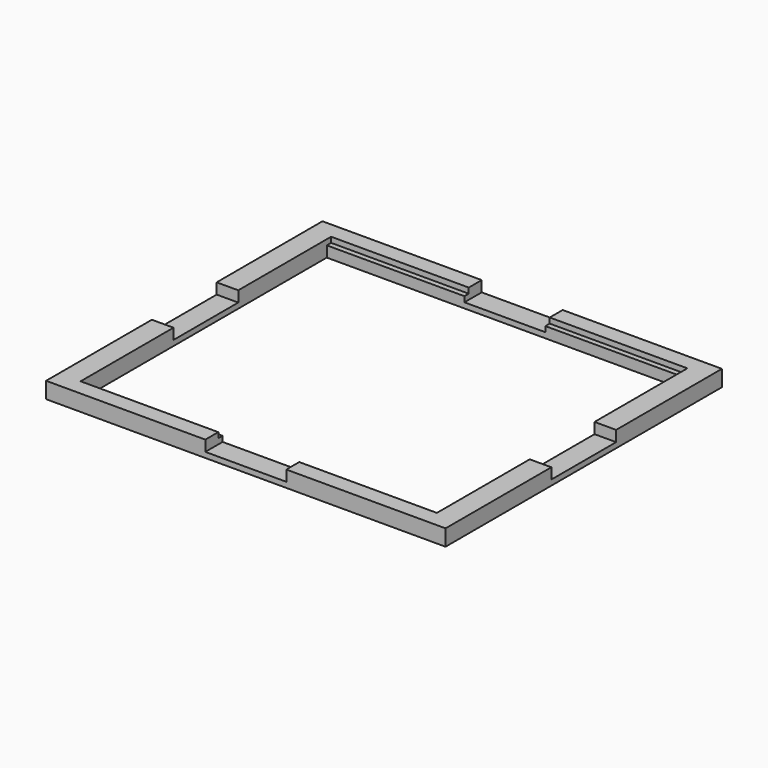
from build123d import *

# Parameters (mm, degrees)
F0_W     = 74
F0_H     = 64
F0_W_2   = 68
F0_H_2   = 58
F0_W_3   = 66
F0_H_3   = 56
F1_DEPTH = 2
F2_W     = 74
F2_H     = 64
F3_DEPTH = 1
F4_W     = 15
F4_H     = 6.5584733043
F4_H_2   = 3
F4_H_3   = 6.1532862581
F4_W_2   = 4
F4_H_4   = 15
F4_W_3   = 1.5584733043
F4_W_4   = 10.1532862581
F5_DEPTH = 2


with BuildPart() as f1:
    # F0 (on Top) → F1 (new body)
    with BuildSketch(Plane.XY):
        with Locations((-34, -29)):
            Rectangle(F0_W, F0_H)
        with Locations((-34, -29)):
            Rectangle(F0_W_2, F0_H_2, mode=Mode.SUBTRACT)
        with Locations((-34, -29)):
            Rectangle(F0_W_2, F0_H_2)
        with Locations((-34, -29)):
            Rectangle(F0_W_3, F0_H_3, mode=Mode.SUBTRACT)
    extrude(amount=F1_DEPTH)

    # F2 (on face) → F3 (join)
    with BuildSketch(Plane.XY.offset(2)):
        with Locations((-34, -29)):
            Rectangle(F2_W, F2_H)
        Polygon((-67, 0), (-1, 0), (-1, -1), (-1, -57), (-1, -58), (-67, -58), (-67, -57), (-67, -1), align=None, mode=Mode.SUBTRACT)
    extrude(amount=F3_DEPTH)

    # F4 (on face) → F5 (cut)
    with BuildSketch(Plane.XY.offset(3)):
        with Locations((-34, 6.2792366521)):
            Rectangle(F4_W, F4_H)
        with Locations((-34, 1.5)):
            Rectangle(F4_W, F4_H_2)
        with Locations((-34, -3.0766431291)):
            Rectangle(F4_W, F4_H_3)
        with Locations((1, -29)):
            Rectangle(F4_W_2, F4_H_4)
        with Locations((3.7792366521, -29)):
            Rectangle(F4_W_3, F4_H_4)
        with Locations((-6.0766431291, -29)):
            Rectangle(F4_W_4, F4_H_4)
        with Locations((-34, -59.5)):
            Rectangle(F4_W, F4_H_2)
        with Locations((-34, -54.9233568709)):
            Rectangle(F4_W, F4_H_3)
        with Locations((-34, -64.2792366521)):
            Rectangle(F4_W, F4_H)
        with Locations((-61.9233568709, -29)):
            Rectangle(F4_W_4, F4_H_4)
        with Locations((-69, -29)):
            Rectangle(F4_W_2, F4_H_4)
        with Locations((-71.7792366521, -29)):
            Rectangle(F4_W_3, F4_H_4)
    extrude(amount=-F5_DEPTH, mode=Mode.SUBTRACT)


solid = f1.part
